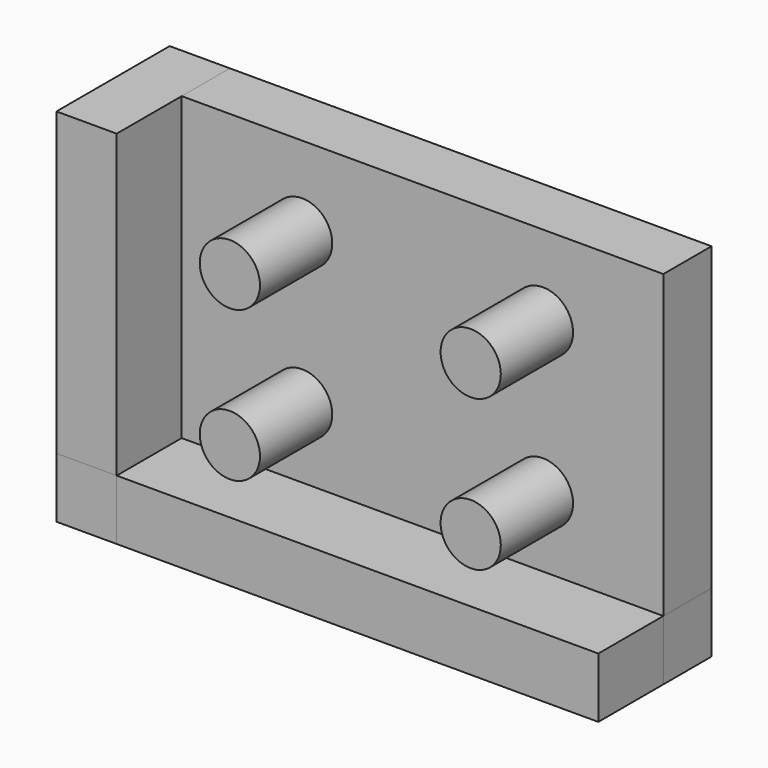
from build123d import *

# Parameters (mm, degrees)
F0_W      = 160
F0_H      = 100
F1_DEPTH  = 20
F3_W      = 27
F3_H      = 100
F4_DEPTH  = 20
F5_DEPTH  = 20
F6_R      = 10
F7_DEPTH  = 30
F9_W      = 160
F9_H      = 27
F10_DEPTH = 20
F11_DEPTH = 20
F12_DEPTH = 20
F13_DEPTH = 20


with BuildPart() as f1:
    # F0 (on Front) → F1 (new body)
    with BuildSketch(Plane.XZ):
        Rectangle(F0_W, F0_H)
    extrude(amount=-F1_DEPTH)

    # F6 (on face) → F7 (join)
    with BuildSketch(Plane.XZ):
        with Locations((-40, -26.8495120108)):
            Circle(F6_R)
        with Locations((-40, 23.1504879892)):
            Circle(F6_R)
        with Locations((40, -26.8495120108)):
            Circle(F6_R)
        with Locations((40, 23.1504879892)):
            Circle(F6_R)
    extrude(amount=F7_DEPTH)


with BuildPart() as f4:
    # F3 (on offset) → F4 (new body)
    with BuildSketch(Plane.YZ.offset(-80)):
        with Locations((-13.5, 0)):
            Rectangle(F3_W, F3_H)
    extrude(amount=-F4_DEPTH)

    # F5 (add): faces of the model
    f5_faces = [f4.faces().sort_by_distance(p)[0] for p in [
        (-90, -27, 0),
        (-90, 0, 0),
    ]]
    extrude(f5_faces, amount=-F5_DEPTH, dir=(0, -1, 0))


with BuildPart() as f10:
    # F9 (on offset) → F10 (new body)
    with BuildSketch(Plane.XY.offset(-50)):
        with Locations((0, -13.5)):
            Rectangle(F9_W, F9_H)
    extrude(amount=-F10_DEPTH)


with BuildPart() as f11:
    # F11 (new, through all): a face of the model
    f11_faces = [f10.part.faces().sort_by_distance(p)[0] for p in [
        (0, 0, -60),
    ]]
    extrude(f11_faces, amount=F11_DEPTH)


with BuildPart() as f12:
    # F12 (new, through all): a face of the model
    f12_faces = [f10.part.faces().sort_by_distance(p)[0] for p in [
        (-80, -13.5, -60),
    ]]
    extrude(f12_faces, amount=F12_DEPTH)


with BuildPart() as f13:
    # F13 (new, through all): a face of the model
    f13_faces = [f11.part.faces().sort_by_distance(p)[0] for p in [
        (-80, 10, -60),
    ]]
    extrude(f13_faces, amount=F13_DEPTH)


solid = Compound([f1.part, f4.part, f10.part, f11.part, f12.part, f13.part])
